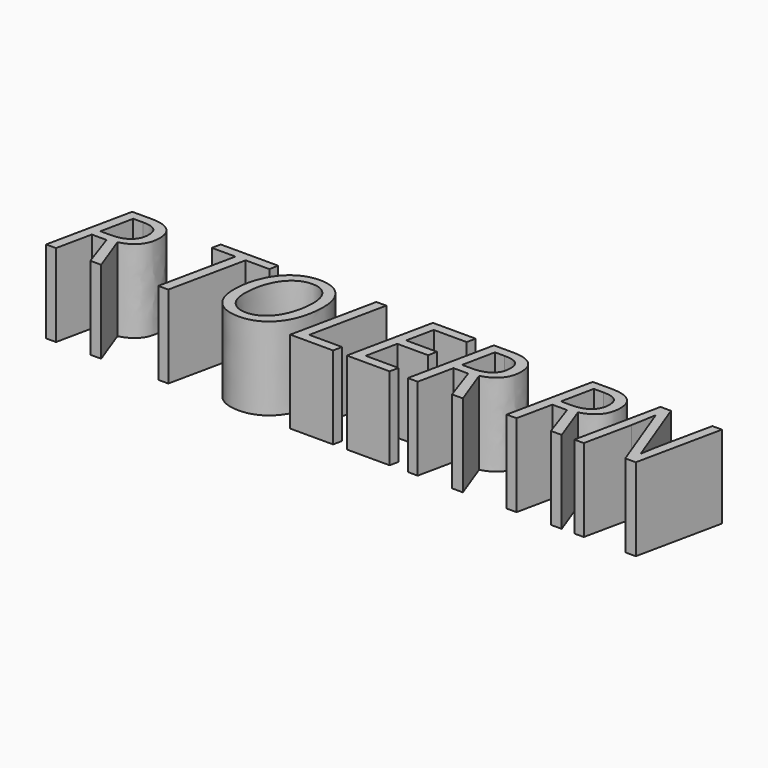
from build123d import *

# Parameters (mm, degrees)
F0_TEXT_SIZE = 36.6214105491
F1_DEPTH     = 25.4


# Not quite as in the source:
# - Text() gives the source's letters only with a copy of the font that has no kerning and outlines rounded to 1/6400 em; it was checked with that copy


with BuildPart() as f1:
    # F0 (on Top) → F1 (new body)
    with BuildSketch(Plane.XY):
        with Locations((-30.7980530451, -14.0557672017)):
            Text('R TOLER RN', F0_TEXT_SIZE, font='Open Sans', font_style=FontStyle.ITALIC, text_align=(TextAlign.LEFT, TextAlign.BOTTOM))
    extrude(amount=F1_DEPTH)


solid = f1.part
